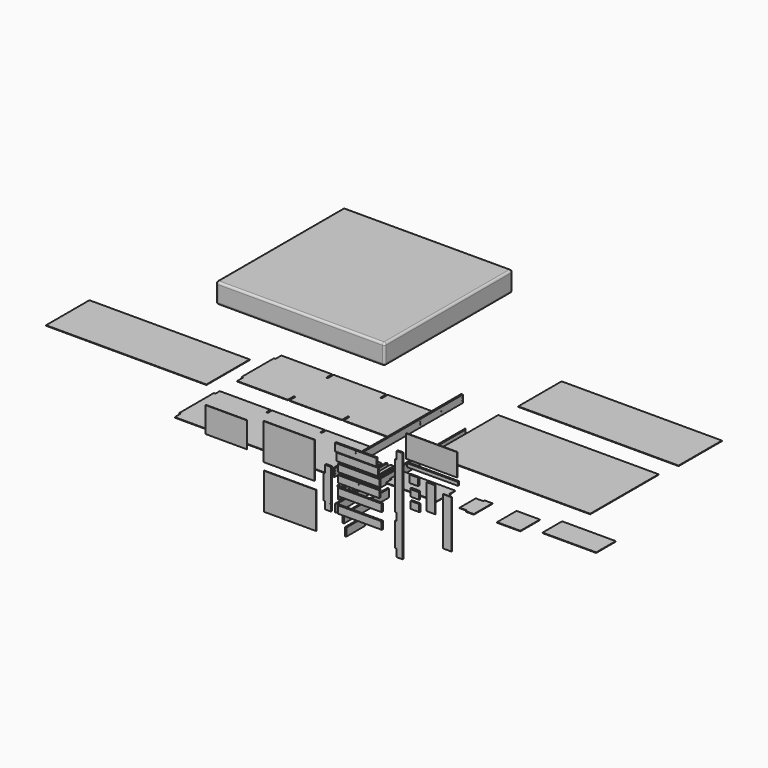
from build123d import *

# Parameters (mm, degrees)
F1_DEPTH   = 19.05
F2_D       = 6.35
F4_D       = 6.35
F4_DEPTH   = 25.4
F4_TIP     = 1.9077324654
F5_D       = 6.35
F5_DEPTH   = 25.4
F5_TIP     = 1.9077324654
F6_D       = 6.35
F6_DEPTH   = 25.4
F6_TIP     = 1.9077324654
F7_D       = 6.35
F7_DEPTH   = 25.4
F7_TIP     = 1.9077324654
F9_D       = 6.35
F9_DEPTH   = 25.4
F9_TIP     = 1.9077324654
F10_D      = 6.35
F10_DEPTH  = 25.4
F10_TIP    = 1.9077324654
F11_D      = 6.35
F11_DEPTH  = 25.4
F11_TIP    = 1.9077324654
F12_D      = 6.35
F12_DEPTH  = 25.4
F12_TIP    = 1.9077324654
F13_D      = 3.302
F13_DEPTH  = 25.4
F13_TIP    = 0.992020882
F14_D      = 3.302
F14_DEPTH  = 25.4
F14_TIP    = 0.992020882
F15_W      = 520.7
F15_H      = 88.9
F16_DEPTH  = 19.05
F17_D      = 6.35
F18_D      = 6.35
F20_D      = 6.35
F20_DEPTH  = 25.4
F20_TIP    = 1.9077324654
F21_D      = 6.35
F21_DEPTH  = 25.4
F21_TIP    = 1.9077324654
F23_D      = 6.35
F23_DEPTH  = 25.4
F23_TIP    = 1.9077324654
F24_D      = 6.35
F24_DEPTH  = 25.4
F24_TIP    = 1.9077324654
F25_D      = 6.35
F26_D      = 6.35
F27_W      = 520.7
F27_H      = 88.9
F28_DEPTH  = 19.05
F30_D      = 6.35
F30_DEPTH  = 25.4
F30_TIP    = 1.9077324654
F31_D      = 6.35
F31_DEPTH  = 25.4
F31_TIP    = 1.9077324654
F33_D      = 6.35
F33_DEPTH  = 25.4
F33_TIP    = 1.9077324654
F34_D      = 6.35
F34_DEPTH  = 25.4
F34_TIP    = 1.9077324654
F36_W      = 41.275
F36_H      = 606.425
F37_DEPTH  = 19.05
F36_H_2    = 628.65
F38_DEPTH  = 19.05
F40_D      = 6.35
F40_DEPTH  = 25.4
F40_TIP    = 1.9077324654
F41_D      = 6.35
F41_DEPTH  = 25.4
F41_TIP    = 1.9077324654
F43_D      = 6.35
F43_DEPTH  = 25.4
F43_TIP    = 1.9077324654
F44_D      = 6.35
F44_DEPTH  = 25.4
F44_TIP    = 1.9077324654
F46_D      = 6.35
F46_DEPTH  = 25.4
F46_TIP    = 1.9077324654
F47_D      = 6.35
F47_DEPTH  = 25.4
F47_TIP    = 1.9077324654
F49_D      = 6.35
F49_DEPTH  = 25.4
F49_TIP    = 1.9077324654
F50_D      = 6.35
F50_DEPTH  = 25.4
F50_TIP    = 1.9077324654
F51_W      = 1917.7
F51_H      = 88.9
F52_DEPTH  = 19.05
F53_D      = 6.35
F54_D      = 6.35
F55_D      = 3.302
F56_D      = 3.302
F57_D      = 6.35
F58_D      = 6.35
F59_D      = 6.35
F60_D      = 6.35
F61_D      = 6.35
F62_D      = 6.35
F63_D      = 3.302
F64_D      = 3.302
F65_W      = 606.425
F65_H      = 431.8
F66_DEPTH  = 6.35
F67_W      = 622.3
F67_H      = 431.8
F68_DEPTH  = 6.35
F70_DEPTH  = 6.35
F71_W      = 715.9752
F71_H      = 95.25
F72_DEPTH  = 17.4752
F73_SIZE   = 17.47519
F74_W      = 1952.6504
F74_H      = 95.25
F75_DEPTH  = 17.4752
F76_SIZE   = 17.47519
F77_SIZE   = 17.47519
F78_W      = 495.3
F78_H      = 6.35
F79_DEPTH  = 12.7
F80_W      = 495.3
F80_H      = 82.55
F81_DEPTH  = 19.05
F83_D      = 6.35
F83_DEPTH  = 25.4
F83_TIP    = 1.9077324654
F84_D      = 6.35
F84_DEPTH  = 25.4
F84_TIP    = 1.9077324654
F86_D      = 6.35
F86_DEPTH  = 25.4
F86_TIP    = 1.9077324654
F87_D      = 5.334
F88_D      = 5.334
F90_DEPTH  = 6.35
F91_W      = 673.1
F91_H      = 95.25
F92_DEPTH  = 17.4752
F93_W      = 495.3
F93_H      = 304.8
F94_DEPTH  = 6.35
F95_W      = 1917.7
F95_H      = 1022.35
F96_DEPTH  = 6.35
F98_DEPTH  = 9.525
F100_D     = 6.35
F100_DEPTH = 25.4
F100_TIP   = 1.9077324654
F101_D     = 6.35
F101_DEPTH = 25.4
F101_TIP   = 1.9077324654
F102_D     = 6.35
F102_DEPTH = 25.4
F102_TIP   = 1.9077324654
F103_W     = 101.6
F103_H     = 88.9
F104_DEPTH = 19.05
F106_D     = 6.35
F106_DEPTH = 25.4
F106_TIP   = 1.9077324654
F108_D     = 6.35
F108_DEPTH = 25.4
F108_TIP   = 1.9077324654
F109_W     = 2019.3
F109_H     = 1917.7
F110_DEPTH = 241.3
F111_R     = 25.4
F113_D     = 6.35
F113_DEPTH = 25.4
F113_TIP   = 1.9077324654
F114_D     = 6.35
F114_DEPTH = 25.4
F114_TIP   = 1.9077324654
F115_W     = 1917.7
F115_H     = 647.7
F116_DEPTH = 6.35
F118_DEPTH = 6.35
F120_DEPTH = 6.35
F121_W     = 279.4
F121_H     = 95.25
F122_DEPTH = 17.4752
F123_W     = 279.4
F123_H     = 292.1
F124_DEPTH = 6.35
F125_W     = 641.35
F125_H     = 292.1
F126_DEPTH = 6.35
F80_H_2    = 6.35
F127_DEPTH = 12.7
F78_H_2    = 82.55
F128_DEPTH = 19.05
F129_D     = 6.35
F130_D     = 6.35
F132_D     = 6.35
F132_DEPTH = 25.4
F132_TIP   = 1.9077324654
F134_D     = 6.35
F134_DEPTH = 25.4
F134_TIP   = 1.9077324654
F135_W     = 495.3
F135_H     = 88.9
F136_DEPTH = 19.05
F138_D     = 6.35
F138_DEPTH = 25.4
F138_TIP   = 1.9077324654
F140_D     = 6.35
F140_DEPTH = 25.4
F140_TIP   = 1.9077324654
F141_W     = 495.3
F141_H     = 88.9
F142_DEPTH = 19.05
F143_D     = 6.35
F144_D     = 6.35
F145_D     = 6.35
F145_DEPTH = 25.4
F145_TIP   = 1.9077324654
F147_D     = 6.35
F147_DEPTH = 25.4
F147_TIP   = 1.9077324654
F149_D     = 6.35
F149_DEPTH = 25.4
F149_TIP   = 1.9077324654
F150_W     = 101.6
F150_H     = 76.2
F151_DEPTH = 19.05
F150_H_2   = 6.35
F152_DEPTH = 12.7
F153_DEPTH = 12.7
F155_D     = 6.35
F155_DEPTH = 25.4
F155_TIP   = 1.9077324654
F157_D     = 6.35
F157_DEPTH = 25.4
F157_TIP   = 1.9077324654
F159_D     = 6.35
F159_DEPTH = 25.4
F159_TIP   = 1.9077324654
F161_D     = 6.35
F161_DEPTH = 25.4
F161_TIP   = 1.9077324654
F162_W     = 101.6
F162_H     = 82.55
F163_DEPTH = 19.05
F162_H_2   = 6.35
F164_DEPTH = 12.7
F166_D     = 6.35
F166_DEPTH = 25.4
F166_TIP   = 1.9077324654
F168_D     = 6.35
F168_DEPTH = 25.4
F168_TIP   = 1.9077324654
F169_W     = 606.425
F169_H     = 41.275
F170_DEPTH = 19.05
F172_D     = 6.35
F172_DEPTH = 25.4
F172_TIP   = 1.9077324654
F174_D     = 6.35
F174_DEPTH = 25.4
F174_TIP   = 1.9077324654
F175_W     = 606.425
F175_H     = 266.7
F176_DEPTH = 6.35
F177_W     = 101.6
F177_H     = 304.8
F178_DEPTH = 6.35
F179_W     = 101.6
F179_H     = 571.5
F180_DEPTH = 6.35
F181_W     = 1917.7
F181_H     = 647.7
F182_DEPTH = 6.35


# Not quite as in the source:
# - a fillet or chamfer is up to 0.001 mm smaller than in the source, because OpenCascade refuses the exact size
# - a feature names something its author has since deleted; it is built from what else it names


with BuildPart() as f1:
    # F0 (on Front) → F1 (new body)
    with BuildSketch(Plane.XZ):
        Polygon((44.0972222222, -217.6638888889), (44.0972222222, 252.2361111111), (-25.7527777778, 252.2361111111), (-25.7527777778, 163.3361111111), (-44.8027777778, 163.3361111111), (-44.8027777778, -128.7638888889), (-25.7527777778, -128.7638888889), (-25.7527777778, -217.6638888889), align=None)
    extrude(amount=F1_DEPTH)

    # F2 (through all)
    with Locations(Plane(origin=(0, 0, 0), x_dir=(1, 0, 0), z_dir=(0, 1, 0))):
        with Locations((36.1597222222, 138.2888888889)):
            Hole(F2_D / 2)

    # F4
    with Locations(Plane.YZ.offset(44.0972222222)):
        with Locations((-9.525, -189.0888888889)):
            Hole(F4_D / 2, depth=F4_DEPTH)
            with Locations((0, 0, -(F4_DEPTH + F4_TIP / 2))):  # 118° drill point
                Cone(0, F4_D / 2, F4_TIP, mode=Mode.SUBTRACT)

    # F5
    with Locations(Plane.YZ.offset(44.0972222222)):
        with Locations((-9.525, -157.3388888889)):
            Hole(F5_D / 2, depth=F5_DEPTH)
            with Locations((0, 0, -(F5_DEPTH + F5_TIP / 2))):  # 118° drill point
                Cone(0, F5_D / 2, F5_TIP, mode=Mode.SUBTRACT)

    # F6
    with Locations(Plane.YZ.offset(44.0972222222)):
        with Locations((-9.525, 223.6611111111)):
            Hole(F6_D / 2, depth=F6_DEPTH)
            with Locations((0, 0, -(F6_DEPTH + F6_TIP / 2))):  # 118° drill point
                Cone(0, F6_D / 2, F6_TIP, mode=Mode.SUBTRACT)

    # F7
    with Locations(Plane.YZ.offset(44.0972222222)):
        with Locations((-9.525, 191.9111111111)):
            Hole(F7_D / 2, depth=F7_DEPTH)
            with Locations((0, 0, -(F7_DEPTH + F7_TIP / 2))):  # 118° drill point
                Cone(0, F7_D / 2, F7_TIP, mode=Mode.SUBTRACT)

    # F9
    with Locations(Plane(origin=(-25.7527777778, 0, 0), x_dir=(0, -1, 0), z_dir=(-1, 0, 0))):
        with Locations((9.525, -189.0888888889)):
            Hole(F9_D / 2, depth=F9_DEPTH)
            with Locations((0, 0, -(F9_DEPTH + F9_TIP / 2))):  # 118° drill point
                Cone(0, F9_D / 2, F9_TIP, mode=Mode.SUBTRACT)

    # F10
    with Locations(Plane(origin=(-25.7527777778, 0, 0), x_dir=(0, -1, 0), z_dir=(-1, 0, 0))):
        with Locations((9.525, -157.3388888889)):
            Hole(F10_D / 2, depth=F10_DEPTH)
            with Locations((0, 0, -(F10_DEPTH + F10_TIP / 2))):  # 118° drill point
                Cone(0, F10_D / 2, F10_TIP, mode=Mode.SUBTRACT)

    # F11
    with Locations(Plane(origin=(-25.7527777778, 0, 0), x_dir=(0, -1, 0), z_dir=(-1, 0, 0))):
        with Locations((9.525, 191.9111111111)):
            Hole(F11_D / 2, depth=F11_DEPTH)
            with Locations((0, 0, -(F11_DEPTH + F11_TIP / 2))):  # 118° drill point
                Cone(0, F11_D / 2, F11_TIP, mode=Mode.SUBTRACT)

    # F12
    with Locations(Plane(origin=(-25.7527777778, 0, 0), x_dir=(0, -1, 0), z_dir=(-1, 0, 0))):
        with Locations((9.525, 223.6611111111)):
            Hole(F12_D / 2, depth=F12_DEPTH)
            with Locations((0, 0, -(F12_DEPTH + F12_TIP / 2))):  # 118° drill point
                Cone(0, F12_D / 2, F12_TIP, mode=Mode.SUBTRACT)

    # F13
    with Locations(Plane(origin=(-25.7527777778, 0, 0), x_dir=(0, -1, 0), z_dir=(-1, 0, 0))):
        with Locations((9.525, -173.2138888889)):
            Hole(F13_D / 2, depth=F13_DEPTH)
            with Locations((0, 0, -(F13_DEPTH + F13_TIP / 2))):  # 118° drill point
                Cone(0, F13_D / 2, F13_TIP, mode=Mode.SUBTRACT)

    # F14
    with Locations(Plane(origin=(-25.7527777778, 0, 0), x_dir=(0, -1, 0), z_dir=(-1, 0, 0))):
        with Locations((9.525, 207.7861111111)):
            Hole(F14_D / 2, depth=F14_DEPTH)
            with Locations((0, 0, -(F14_DEPTH + F14_TIP / 2))):  # 118° drill point
                Cone(0, F14_D / 2, F14_TIP, mode=Mode.SUBTRACT)


with BuildPart() as f16:
    # F15 (on Front) → F16 (new body)
    with BuildSketch(Plane.XZ):
        with Locations((392.2159543753, -168.203163892)):
            Rectangle(F15_W, F15_H)
    extrude(amount=F16_DEPTH)

    # F17 (through all)
    with Locations(Plane(origin=(0, 0, 0), x_dir=(1, 0, 0), z_dir=(0, 1, 0))):
        with Locations((139.8161543753, 133.278163892)):
            Hole(F17_D / 2)

    # F18 (through all)
    with Locations(Plane(origin=(0, 0, 0), x_dir=(1, 0, 0), z_dir=(0, 1, 0))):
        with Locations((644.6157543753, 133.278163892)):
            Hole(F18_D / 2)

    # F20
    with Locations(Plane.YZ.offset(652.5659543753)):
        with Locations((-9.525, -152.328163892)):
            Hole(F20_D / 2, depth=F20_DEPTH)
            with Locations((0, 0, -(F20_DEPTH + F20_TIP / 2))):  # 118° drill point
                Cone(0, F20_D / 2, F20_TIP, mode=Mode.SUBTRACT)

    # F21
    with Locations(Plane.YZ.offset(652.5659543753)):
        with Locations((-9.525, -184.078163892)):
            Hole(F21_D / 2, depth=F21_DEPTH)
            with Locations((0, 0, -(F21_DEPTH + F21_TIP / 2))):  # 118° drill point
                Cone(0, F21_D / 2, F21_TIP, mode=Mode.SUBTRACT)

    # F23
    with Locations(Plane(origin=(131.8659543753, 0, 0), x_dir=(0, -1, 0), z_dir=(-1, 0, 0))):
        with Locations((9.525, -152.328163892)):
            Hole(F23_D / 2, depth=F23_DEPTH)
            with Locations((0, 0, -(F23_DEPTH + F23_TIP / 2))):  # 118° drill point
                Cone(0, F23_D / 2, F23_TIP, mode=Mode.SUBTRACT)

    # F24
    with Locations(Plane(origin=(131.8659543753, 0, 0), x_dir=(0, -1, 0), z_dir=(-1, 0, 0))):
        with Locations((9.525, -184.078163892)):
            Hole(F24_D / 2, depth=F24_DEPTH)
            with Locations((0, 0, -(F24_DEPTH + F24_TIP / 2))):  # 118° drill point
                Cone(0, F24_D / 2, F24_TIP, mode=Mode.SUBTRACT)

    # F25 (through all)
    with Locations(Plane(origin=(0, 0, 0), x_dir=(1, 0, 0), z_dir=(0, 1, 0))):
        with Locations((392.2159543753, 136.453163892)):
            Hole(F25_D / 2)

    # F26 (through all)
    with Locations(Plane(origin=(0, 0, 0), x_dir=(1, 0, 0), z_dir=(0, 1, 0))):
        with Locations((392.2159543753, 152.328163892)):
            Hole(F26_D / 2)


with BuildPart() as f28:
    # F27 (on Front) → F28 (new body)
    with BuildSketch(Plane.XZ):
        with Locations((390.0367697954, 17.3669979692)):
            Rectangle(F27_W, F27_H)
    extrude(amount=F28_DEPTH)

    # F30
    with Locations(Plane.YZ.offset(650.3867697954)):
        with Locations((-9.525, 33.2419979692)):
            Hole(F30_D / 2, depth=F30_DEPTH)
            with Locations((0, 0, -(F30_DEPTH + F30_TIP / 2))):  # 118° drill point
                Cone(0, F30_D / 2, F30_TIP, mode=Mode.SUBTRACT)

    # F31
    with Locations(Plane.YZ.offset(650.3867697954)):
        with Locations((-9.525, 1.4919979692)):
            Hole(F31_D / 2, depth=F31_DEPTH)
            with Locations((0, 0, -(F31_DEPTH + F31_TIP / 2))):  # 118° drill point
                Cone(0, F31_D / 2, F31_TIP, mode=Mode.SUBTRACT)

    # F33
    with Locations(Plane(origin=(129.6867697954, 0, 0), x_dir=(0, -1, 0), z_dir=(-1, 0, 0))):
        with Locations((9.525, 33.2419979692)):
            Hole(F33_D / 2, depth=F33_DEPTH)
            with Locations((0, 0, -(F33_DEPTH + F33_TIP / 2))):  # 118° drill point
                Cone(0, F33_D / 2, F33_TIP, mode=Mode.SUBTRACT)

    # F34
    with Locations(Plane(origin=(129.6867697954, 0, 0), x_dir=(0, -1, 0), z_dir=(-1, 0, 0))):
        with Locations((9.525, 1.4919979692)):
            Hole(F34_D / 2, depth=F34_DEPTH)
            with Locations((0, 0, -(F34_DEPTH + F34_TIP / 2))):  # 118° drill point
                Cone(0, F34_D / 2, F34_TIP, mode=Mode.SUBTRACT)


with BuildPart() as f37:
    # F36 (on face) → F37 (new body)
    with BuildSketch(Plane.XY):
        with Locations((65.2231872082, 383.8816340816)):
            Rectangle(F36_W, F36_H)
    extrude(amount=F37_DEPTH)

    # F43
    with Locations(Plane.XZ.offset(-80.6691340816)):
        with Locations((73.1606872082, 9.525)):
            Hole(F43_D / 2, depth=F43_DEPTH)
            with Locations((0, 0, -(F43_DEPTH + F43_TIP / 2))):  # 118° drill point
                Cone(0, F43_D / 2, F43_TIP, mode=Mode.SUBTRACT)

    # F44
    with Locations(Plane.XZ.offset(-80.6691340816)):
        with Locations((57.2856872082, 9.525)):
            Hole(F44_D / 2, depth=F44_DEPTH)
            with Locations((0, 0, -(F44_DEPTH + F44_TIP / 2))):  # 118° drill point
                Cone(0, F44_D / 2, F44_TIP, mode=Mode.SUBTRACT)

    # F46
    with Locations(Plane(origin=(0, 687.0941340816, 0), x_dir=(-1, 0, 0), z_dir=(0, 1, 0))):
        with Locations((-73.1606872082, 9.525)):
            Hole(F46_D / 2, depth=F46_DEPTH)
            with Locations((0, 0, -(F46_DEPTH + F46_TIP / 2))):  # 118° drill point
                Cone(0, F46_D / 2, F46_TIP, mode=Mode.SUBTRACT)

    # F47
    with Locations(Plane(origin=(0, 687.0941340816, 0), x_dir=(-1, 0, 0), z_dir=(0, 1, 0))):
        with Locations((-57.2856872082, 9.525)):
            Hole(F47_D / 2, depth=F47_DEPTH)
            with Locations((0, 0, -(F47_DEPTH + F47_TIP / 2))):  # 118° drill point
                Cone(0, F47_D / 2, F47_TIP, mode=Mode.SUBTRACT)


with BuildPart() as f38:
    # F36 (on face) → F38 (new body)
    with BuildSketch(Plane.XY):
        with Locations((191.2130686522, 397.9515534163)):
            Rectangle(F36_W, F36_H_2)
    extrude(amount=F38_DEPTH)

    # F40
    with Locations(Plane.XZ.offset(-83.6265534163)):
        with Locations((183.2755686522, 9.525)):
            Hole(F40_D / 2, depth=F40_DEPTH)
            with Locations((0, 0, -(F40_DEPTH + F40_TIP / 2))):  # 118° drill point
                Cone(0, F40_D / 2, F40_TIP, mode=Mode.SUBTRACT)

    # F41
    with Locations(Plane.XZ.offset(-83.6265534163)):
        with Locations((199.1505686522, 9.525)):
            Hole(F41_D / 2, depth=F41_DEPTH)
            with Locations((0, 0, -(F41_DEPTH + F41_TIP / 2))):  # 118° drill point
                Cone(0, F41_D / 2, F41_TIP, mode=Mode.SUBTRACT)

    # F49
    with Locations(Plane(origin=(0, 712.2765534163, 0), x_dir=(-1, 0, 0), z_dir=(0, 1, 0))):
        with Locations((-183.2755686522, 10.0011052564)):
            Hole(F49_D / 2, depth=F49_DEPTH)
            with Locations((0, 0, -(F49_DEPTH + F49_TIP / 2))):  # 118° drill point
                Cone(0, F49_D / 2, F49_TIP, mode=Mode.SUBTRACT)

    # F50
    with Locations(Plane(origin=(0, 712.2765534163, 0), x_dir=(-1, 0, 0), z_dir=(0, 1, 0))):
        with Locations((-199.1505686522, 9.525)):
            Hole(F50_D / 2, depth=F50_DEPTH)
            with Locations((0, 0, -(F50_DEPTH + F50_TIP / 2))):  # 118° drill point
                Cone(0, F50_D / 2, F50_TIP, mode=Mode.SUBTRACT)


with BuildPart() as f52:
    # F51 (on Right) → F52 (new body)
    with BuildSketch(Plane.YZ):
        with Locations((1025.7683731079, 146.691538465)):
            Rectangle(F51_W, F51_H)
    extrude(amount=F52_DEPTH)

    # F53 (through all)
    with Locations(Plane(origin=(0, 0, 0), x_dir=(0, 1, 0), z_dir=(-1, 0, 0))):
        with Locations((76.4433731079, -162.566538465)):
            Hole(F53_D / 2)

    # F54 (through all)
    with Locations(Plane(origin=(0, 0, 0), x_dir=(0, 1, 0), z_dir=(-1, 0, 0))):
        with Locations((76.4433731079, -130.816538465)):
            Hole(F54_D / 2)

    # F55 (through all)
    with Locations(Plane(origin=(0, 0, 0), x_dir=(0, 1, 0), z_dir=(-1, 0, 0))):
        with Locations((76.4433731079, -146.691538465)):
            Hole(F55_D / 2)

    # F56 (through all)
    with Locations(Plane(origin=(0, 0, 0), x_dir=(0, 1, 0), z_dir=(-1, 0, 0))):
        with Locations((1975.0933731079, -146.691538465)):
            Hole(F56_D / 2)

    # F57 (through all)
    with Locations(Plane(origin=(0, 0, 0), x_dir=(0, 1, 0), z_dir=(-1, 0, 0))):
        with Locations((1975.0933731079, -162.566538465)):
            Hole(F57_D / 2)

    # F58 (through all)
    with Locations(Plane(origin=(0, 0, 0), x_dir=(0, 1, 0), z_dir=(-1, 0, 0))):
        with Locations((1975.0933731079, -130.816538465)):
            Hole(F58_D / 2)

    # F59 (through all)
    with Locations(Plane(origin=(0, 0, 0), x_dir=(0, 1, 0), z_dir=(-1, 0, 0))):
        with Locations((1349.6183731079, -162.566538465)):
            Hole(F59_D / 2)

    # F60 (through all)
    with Locations(Plane(origin=(0, 0, 0), x_dir=(0, 1, 0), z_dir=(-1, 0, 0))):
        with Locations((1349.6183731079, -130.816538465)):
            Hole(F60_D / 2)

    # F61 (through all)
    with Locations(Plane(origin=(0, 0, 0), x_dir=(0, 1, 0), z_dir=(-1, 0, 0))):
        with Locations((701.9183731079, -162.566538465)):
            Hole(F61_D / 2)

    # F62 (through all)
    with Locations(Plane(origin=(0, 0, 0), x_dir=(0, 1, 0), z_dir=(-1, 0, 0))):
        with Locations((701.9183731079, -130.816538465)):
            Hole(F62_D / 2)

    # F63 (through all)
    with Locations(Plane(origin=(0, 0, 0), x_dir=(0, 1, 0), z_dir=(-1, 0, 0))):
        with Locations((701.9183731079, -146.691538465)):
            Hole(F63_D / 2)

    # F64 (through all)
    with Locations(Plane(origin=(0, 0, 0), x_dir=(0, 1, 0), z_dir=(-1, 0, 0))):
        with Locations((1349.6183731079, -146.691538465)):
            Hole(F64_D / 2)

    # F87 (through all)
    with Locations(Plane(origin=(0, 0, 0), x_dir=(0, 1, 0), z_dir=(-1, 0, 0))):
        with Locations((1662.3431731079, -146.691538465)):
            Hole(F87_D / 2)

    # F88 (through all)
    with Locations(Plane(origin=(0, 0, 0), x_dir=(0, 1, 0), z_dir=(-1, 0, 0))):
        with Locations((389.1808731079, -146.691538465)):
            Hole(F88_D / 2)


with BuildPart() as f66:
    # F65 (on Front) → F66 (new body)
    with BuildSketch(Plane.XZ):
        with Locations((-466.6956380844, 248.3464175232)):
            Rectangle(F65_W, F65_H)
    extrude(amount=F66_DEPTH)


with BuildPart() as f68:
    # F67 (on face) → F68 (new body)
    with BuildSketch(Plane.XZ.offset(6.35)):
        with Locations((-450.0797018051, -268.8254054308)):
            Rectangle(F67_W, F67_H)
    extrude(amount=F68_DEPTH)


with BuildPart() as f70:
    # F69 (on Top) → F70 (new body)
    with BuildSketch(Plane.XY):
        Polygon((-1412.1244818761, 898.8181884059), (-2018.5494818761, 898.8181884059), (-2018.5494818761, 835.3181884059), (-2037.5994818761, 835.3181884059), (-2037.5994818761, 314.6181884059), (-2018.5494818761, 314.6181884059), (-2018.5494818761, 225.7181884059), (-1412.1244818761, 225.7181884059), (-1412.1244818761, 314.6181884059), (-1393.0744818761, 314.6181884059), (-1393.0744818761, 225.7181884059), (-764.4244818761, 225.7181884059), (-764.4244818761, 314.6181884059), (-745.3744818761, 314.6181884059), (-745.3744818761, 225.7181884059), (-138.9494818761, 225.7181884059), (-138.9494818761, 314.6181884059), (-119.8994818761, 314.6181884059), (-119.8994818761, 835.3181884059), (-138.9494818761, 835.3181884059), (-138.9494818761, 898.8181884059), (-745.3744818761, 898.8181884059), (-745.3744818761, 835.3181884059), (-764.4244818761, 835.3181884059), (-764.4244818761, 898.8181884059), (-1393.0744818761, 898.8181884059), (-1393.0744818761, 835.3181884059), (-1412.1244818761, 835.3181884059), align=None)
    extrude(amount=F70_DEPTH)


with BuildPart() as f72:
    # F71 (on Right) → F72 (new body)
    with BuildSketch(Plane.YZ):
        with Locations((501.9332787514, -122.720502317)):
            Rectangle(F71_W, F71_H)
    extrude(amount=F72_DEPTH)

    # F73 (size 17.4752 in the source; OpenCascade refuses exactly that, so slightly less here)
    f73_edges = [f72.edges().sort_by_distance(p)[0] for p in [
        (17.4752, 143.945679, -122.720502),
    ]]
    chamfer(f73_edges, length=F73_SIZE)


with BuildPart() as f75:
    # F74 (on Right) → F75 (new body)
    with BuildSketch(Plane.YZ):
        with Locations((1071.8703280807, -243.98250422)):
            Rectangle(F74_W, F74_H)
    extrude(amount=F75_DEPTH)

    # F76 (size 17.4752 in the source; OpenCascade refuses exactly that, so slightly less here)
    f76_edges = [f75.edges().sort_by_distance(p)[0] for p in [
        (17.4752, 95.545128, -243.982504),
    ]]
    chamfer(f76_edges, length=F76_SIZE)

    # F77 (size 17.4752 in the source; OpenCascade refuses exactly that, so slightly less here)
    f77_edges = [f75.edges().sort_by_distance(p)[0] for p in [
        (17.4752, 2048.195528, -243.982504),
    ]]
    chamfer(f77_edges, length=F77_SIZE)


with BuildPart() as f79:
    # F78 (on Front) → F79 (new body)
    with BuildSketch(Plane.XZ):
        with Locations((375.5939779373, 197.4594274402)):
            Rectangle(F78_W, F78_H)
    extrude(amount=F79_DEPTH)

    # F78 (on Front) → F128 (join)
    with BuildSketch(Plane.XZ):
        with Locations((375.5939779373, 153.0094274402)):
            Rectangle(F78_W, F78_H_2)
    extrude(amount=F128_DEPTH)

    # F129 (through all)
    with Locations(Plane(origin=(0, 0, 0), x_dir=(1, 0, 0), z_dir=(0, 1, 0))):
        with Locations((375.5939779373, -187.9344274402)):
            Hole(F129_D / 2)

    # F130 (through all)
    with Locations(Plane(origin=(0, 0, 0), x_dir=(1, 0, 0), z_dir=(0, 1, 0))):
        with Locations((375.5939779373, -172.0594274402)):
            Hole(F130_D / 2)

    # F132
    with Locations(Plane(origin=(127.9439779373, 0, 0), x_dir=(0, -1, 0), z_dir=(-1, 0, 0))):
        with Locations((9.525, 172.0594274402), (9.525, 140.3094274402)):
            Hole(F132_D / 2, depth=F132_DEPTH)
            with Locations((0, 0, -(F132_DEPTH + F132_TIP / 2))):  # 118° drill point
                Cone(0, F132_D / 2, F132_TIP, mode=Mode.SUBTRACT)

    # F134
    with Locations(Plane.YZ.offset(623.2439779373)):
        with Locations((-9.525, 172.0594274402), (-9.525, 140.3094274402)):
            Hole(F134_D / 2, depth=F134_DEPTH)
            with Locations((0, 0, -(F134_DEPTH + F134_TIP / 2))):  # 118° drill point
                Cone(0, F134_D / 2, F134_TIP, mode=Mode.SUBTRACT)


with BuildPart() as f81:
    # F80 (on Front) → F81 (new body)
    with BuildSketch(Plane.XZ):
        with Locations((375.3500119215, 270.1343170285)):
            Rectangle(F80_W, F80_H)
    extrude(amount=F81_DEPTH)

    # F83
    with Locations(Plane(origin=(127.7000119215, 0, 0), x_dir=(0, -1, 0), z_dir=(-1, 0, 0))):
        with Locations((9.525, 282.8343170285)):
            Hole(F83_D / 2, depth=F83_DEPTH)
            with Locations((0, 0, -(F83_DEPTH + F83_TIP / 2))):  # 118° drill point
                Cone(0, F83_D / 2, F83_TIP, mode=Mode.SUBTRACT)

    # F84
    with Locations(Plane(origin=(127.7000119215, 0, 0), x_dir=(0, -1, 0), z_dir=(-1, 0, 0))):
        with Locations((9.525, 251.0843170285)):
            Hole(F84_D / 2, depth=F84_DEPTH)
            with Locations((0, 0, -(F84_DEPTH + F84_TIP / 2))):  # 118° drill point
                Cone(0, F84_D / 2, F84_TIP, mode=Mode.SUBTRACT)

    # F86
    with Locations(Plane.YZ.offset(623.0000119215)):
        with Locations((-9.525, 282.8343170285)):
            Hole(F86_D / 2, depth=F86_DEPTH)
            with Locations((0, 0, -(F86_DEPTH + F86_TIP / 2))):  # 118° drill point
                Cone(0, F86_D / 2, F86_TIP, mode=Mode.SUBTRACT)

    # F80 (on Front) → F127 (join)
    with BuildSketch(Plane.XZ):
        with Locations((375.3500119215, 225.6843170285)):
            Rectangle(F80_W, F80_H_2)
    extrude(amount=F127_DEPTH)

    # F145
    with Locations(Plane.YZ.offset(623.0000119215)):
        with Locations((-9.525, 251.0843170285)):
            Hole(F145_D / 2, depth=F145_DEPTH)
            with Locations((0, 0, -(F145_DEPTH + F145_TIP / 2))):  # 118° drill point
                Cone(0, F145_D / 2, F145_TIP, mode=Mode.SUBTRACT)


with BuildPart() as f90:
    # F89 (on Top) → F90 (new body)
    with BuildSketch(Plane.XY):
        Polygon((-1412.908935664, 1820.1076601933), (-2019.333935664, 1820.1076601933), (-2019.333935664, 1731.2076601933), (-2038.383935664, 1731.2076601933), (-2038.383935664, 1248.6076601933), (-2019.333935664, 1248.6076601933), (-2019.333935664, 1159.7076601933), (-1412.908935664, 1159.7076601933), (-1412.908935664, 1248.6076601933), (-1393.858935664, 1248.6076601933), (-1393.858935664, 1159.7076601933), (-765.208935664, 1159.7076601933), (-765.208935664, 1248.6076601933), (-746.158935664, 1248.6076601933), (-746.158935664, 1159.7076601933), (-139.733935664, 1159.7076601933), (-139.733935664, 1248.6076601933), (-120.683935664, 1248.6076601933), (-120.683935664, 1731.2076601933), (-139.733935664, 1731.2076601933), (-139.733935664, 1820.1076601933), (-746.158935664, 1820.1076601933), (-746.158935664, 1731.2076601933), (-765.208935664, 1731.2076601933), (-765.208935664, 1820.1076601933), (-1393.858935664, 1820.1076601933), (-1393.858935664, 1731.2076601933), (-1412.908935664, 1731.2076601933), align=None)
    extrude(amount=F90_DEPTH)


with BuildPart() as f92:
    # F91 (on Right) → F92 (new body)
    with BuildSketch(Plane.YZ):
        with Locations((547.2309960085, -398.1397897005)):
            Rectangle(F91_W, F91_H)
    extrude(amount=F92_DEPTH)


with BuildPart() as f94:
    # F93 (on Front) → F94 (new body)
    with BuildSketch(Plane.XZ):
        with Locations((-1218.936782995, 254.6093458474)):
            Rectangle(F93_W, F93_H)
    extrude(amount=F94_DEPTH)


with BuildPart() as f96:
    # F95 (on face) → F96 (new body)
    with BuildSketch(Plane.XY.offset(6.35)):
        with Locations((1280.6541621685, 1624.7996635968)):
            Rectangle(F95_W, F95_H)
    extrude(amount=F96_DEPTH)


with BuildPart() as f98:
    # F97 (on Front) → F98 (new body, symmetric)
    with BuildSketch(Plane.XZ):
        Polygon((823.0462499619, -359.8734816171), (823.0462499619, -448.7734816171), (892.8962499619, -448.7734816171), (892.8962499619, 668.8265183829), (823.0462499619, 668.8265183829), (823.0462499619, 579.9265183829), (803.9962499619, 579.9265183829), (803.9962499619, 478.3265183829), (803.9962499619, 389.4265183829), (803.9962499619, 21.1265183829), (823.0462499619, 21.1265183829), (823.0462499619, -67.7734816171), (803.9962499619, -67.7734816171), (803.9962499619, -359.8734816171), align=None)
    extrude(amount=F98_DEPTH, both=True)

    # F100
    with Locations(Plane.YZ.offset(892.8962499619)):
        with Locations((0, -420.1984816171)):
            Hole(F100_D / 2, depth=F100_DEPTH)
            with Locations((0, 0, -(F100_DEPTH + F100_TIP / 2))):  # 118° drill point
                Cone(0, F100_D / 2, F100_TIP, mode=Mode.SUBTRACT)

    # F101
    with Locations(Plane.YZ.offset(892.8962499619)):
        with Locations((0, -388.4484816171)):
            Hole(F101_D / 2, depth=F101_DEPTH)
            with Locations((0, 0, -(F101_DEPTH + F101_TIP / 2))):  # 118° drill point
                Cone(0, F101_D / 2, F101_TIP, mode=Mode.SUBTRACT)

    # F102
    with Locations(Plane.YZ.offset(892.8962499619)):
        with Locations((0, -7.4484816171), (0, -39.1984816171)):
            Hole(F102_D / 2, depth=F102_DEPTH)
            with Locations((0, 0, -(F102_DEPTH + F102_TIP / 2))):  # 118° drill point
                Cone(0, F102_D / 2, F102_TIP, mode=Mode.SUBTRACT)

    # F113
    with Locations(Plane(origin=(823.0462499619, 0, 0), x_dir=(0, -1, 0), z_dir=(-1, 0, 0))):
        with Locations((0, 640.2515183829), (0, 608.5015183829)):
            Hole(F113_D / 2, depth=F113_DEPTH)
            with Locations((0, 0, -(F113_DEPTH + F113_TIP / 2))):  # 118° drill point
                Cone(0, F113_D / 2, F113_TIP, mode=Mode.SUBTRACT)

    # F114
    with Locations(Plane.YZ.offset(892.8962499619)):
        with Locations((0, 640.2515183829), (0, 608.5015183829)):
            Hole(F114_D / 2, depth=F114_DEPTH)
            with Locations((0, 0, -(F114_DEPTH + F114_TIP / 2))):  # 118° drill point
                Cone(0, F114_D / 2, F114_TIP, mode=Mode.SUBTRACT)

    # F159
    with Locations(Plane(origin=(823.0462499619, 0, 0), x_dir=(0, -1, 0), z_dir=(-1, 0, 0))):
        with Locations((0, -7.4484816171), (0, -39.1984816171)):
            Hole(F159_D / 2, depth=F159_DEPTH)
            with Locations((0, 0, -(F159_DEPTH + F159_TIP / 2))):  # 118° drill point
                Cone(0, F159_D / 2, F159_TIP, mode=Mode.SUBTRACT)

    # F161
    with Locations(Plane(origin=(823.0462499619, 0, 0), x_dir=(0, -1, 0), z_dir=(-1, 0, 0))):
        with Locations((0, -388.4484816171), (0, -420.1984816171)):
            Hole(F161_D / 2, depth=F161_DEPTH)
            with Locations((0, 0, -(F161_DEPTH + F161_TIP / 2))):  # 118° drill point
                Cone(0, F161_D / 2, F161_TIP, mode=Mode.SUBTRACT)


with BuildPart() as f104:
    # F103 (on face) → F104 (new body)
    with BuildSketch(Plane.XZ.offset(9.525)):
        with Locations((1043.4946498871, 439.289823246)):
            Rectangle(F103_W, F103_H)
    extrude(amount=F104_DEPTH)

    # F106
    with Locations(Plane.YZ.offset(1094.2946498871)):
        with Locations((-19.05, 455.164823246), (-19.05, 423.414823246)):
            Hole(F106_D / 2, depth=F106_DEPTH)
            with Locations((0, 0, -(F106_DEPTH + F106_TIP / 2))):  # 118° drill point
                Cone(0, F106_D / 2, F106_TIP, mode=Mode.SUBTRACT)

    # F108
    with Locations(Plane(origin=(992.6946498871, 0, 0), x_dir=(0, -1, 0), z_dir=(-1, 0, 0))):
        with Locations((19.05, 455.164823246), (19.05, 423.414823246)):
            Hole(F108_D / 2, depth=F108_DEPTH)
            with Locations((0, 0, -(F108_DEPTH + F108_TIP / 2))):  # 118° drill point
                Cone(0, F108_D / 2, F108_TIP, mode=Mode.SUBTRACT)


with BuildPart() as f110:
    # F109 (on Top) → F110 (new body)
    with BuildSketch(Plane.XY):
        with Locations((-2145.1758291454, 3216.1710262299)):
            Rectangle(F109_W, F109_H)
    extrude(amount=F110_DEPTH)

    # F111
    f111_edges = [f110.edges().sort_by_distance(p)[0] for p in [
        (-2145.175829, 2257.321026, 241.3),
        (-3154.825829, 2257.321026, 120.65),
        (-3154.825829, 3216.171026, 241.3),
        (-2145.175829, 2257.321026, 0),
        (-3154.825829, 3216.171026, 0),
        (-1135.525829, 2257.321026, 120.65),
        (-1135.525829, 3216.171026, 241.3),
        (-1135.525829, 3216.171026, 0),
        (-1135.525829, 4175.021026, 120.65),
        (-2145.175829, 4175.021026, 241.3),
        (-3154.825829, 4175.021026, 120.65),
        (-2145.175829, 4175.021026, 0),
    ]]
    fillet(f111_edges, radius=F111_R)


with BuildPart() as f116:
    # F115 (on face) → F116 (new body)
    with BuildSketch(Plane.XY.offset(12.7)):
        with Locations((1324.3790087512, 2704.3896711349)):
            Rectangle(F115_W, F115_H)
    extrude(amount=F116_DEPTH)


with BuildPart() as f118:
    # F117 (on Top) → F118 (new body)
    with BuildSketch(Plane.XY):
        Polygon((954.666505909, 701.1590391636), (348.241505909, 701.1590391636), (348.241505909, 612.2590391636), (329.191505909, 612.2590391636), (329.191505909, 510.6590391636), (348.241505909, 510.6590391636), (348.241505909, 421.7590391636), (954.666505909, 421.7590391636), (954.666505909, 510.6590391636), (973.716505909, 510.6590391636), (973.716505909, 612.2590391636), (954.666505909, 612.2590391636), align=None)
    extrude(amount=F118_DEPTH)


with BuildPart() as f120:
    # F119 (on face) → F120 (new body)
    with BuildSketch(Plane.XY.offset(6.35)):
        Polygon((1394.9772543545, 707.9822912931), (1299.7272543545, 707.9822912931), (1299.7272543545, 688.9322912931), (1210.8272543545, 688.9322912931), (1210.8272543545, 447.6322912931), (1299.7272543545, 447.6322912931), (1299.7272543545, 428.5822912931), (1394.9772543545, 428.5822912931), align=None)
    extrude(amount=F120_DEPTH)


with BuildPart() as f122:
    # F121 (on face) → F122 (new body)
    with BuildSketch(Plane.YZ.offset(17.4752)):
        with Locations((362.692411232, -536.618118763)):
            Rectangle(F121_W, F121_H)
    extrude(amount=F122_DEPTH)


with BuildPart() as f124:
    # F123 (on face) → F124 (new body)
    with BuildSketch(Plane.XY.offset(12.7)):
        with Locations((1813.7959793091, 573.3920572281)):
            Rectangle(F123_W, F123_H)
    extrude(amount=F124_DEPTH)


with BuildPart() as f126:
    # F125 (on face) → F126 (new body)
    with BuildSketch(Plane.XY.offset(19.05)):
        with Locations((2465.9060394287, 665.3391359329)):
            Rectangle(F125_W, F125_H)
    extrude(amount=F126_DEPTH)


with BuildPart() as f136:
    # F135 (on face) → F136 (new body)
    with BuildSketch(Plane.XZ.offset(19.05)):
        with Locations((372.6696048737, 393.4240490913)):
            Rectangle(F135_W, F135_H)
    extrude(amount=F136_DEPTH)

    # F138
    with Locations(Plane(origin=(125.0196048737, 0, 0), x_dir=(0, -1, 0), z_dir=(-1, 0, 0))):
        with Locations((28.575, 409.2990490913), (28.575, 377.5490490913)):
            Hole(F138_D / 2, depth=F138_DEPTH)
            with Locations((0, 0, -(F138_DEPTH + F138_TIP / 2))):  # 118° drill point
                Cone(0, F138_D / 2, F138_TIP, mode=Mode.SUBTRACT)

    # F140
    with Locations(Plane.YZ.offset(620.3196048737)):
        with Locations((-28.575, 409.2990490913), (-28.575, 377.5490490913)):
            Hole(F140_D / 2, depth=F140_DEPTH)
            with Locations((0, 0, -(F140_DEPTH + F140_TIP / 2))):  # 118° drill point
                Cone(0, F140_D / 2, F140_TIP, mode=Mode.SUBTRACT)


with BuildPart() as f142:
    # F141 (on face) → F142 (new body)
    with BuildSketch(Plane.XZ.offset(38.1)):
        with Locations((371.7590843201, 502.6594550133)):
            Rectangle(F141_W, F141_H)
    extrude(amount=F142_DEPTH)

    # F143 (through all)
    with Locations(Plane(origin=(0, -38.1, 0), x_dir=(1, 0, 0), z_dir=(0, 1, 0))):
        with Locations((371.7590843201, -534.4094550133)):
            Hole(F143_D / 2)

    # F144 (through all)
    with Locations(Plane(origin=(0, -38.1, 0), x_dir=(1, 0, 0), z_dir=(0, 1, 0))):
        with Locations((371.7590843201, -518.5344550133)):
            Hole(F144_D / 2)

    # F147
    with Locations(Plane.YZ.offset(619.4090843201)):
        with Locations((-47.625, 518.5344550133), (-47.625, 486.7844550133)):
            Hole(F147_D / 2, depth=F147_DEPTH)
            with Locations((0, 0, -(F147_DEPTH + F147_TIP / 2))):  # 118° drill point
                Cone(0, F147_D / 2, F147_TIP, mode=Mode.SUBTRACT)

    # F149
    with Locations(Plane(origin=(124.1090843201, 0, 0), x_dir=(0, -1, 0), z_dir=(-1, 0, 0))):
        with Locations((47.625, 518.5344550133), (47.625, 486.7844550133)):
            Hole(F149_D / 2, depth=F149_DEPTH)
            with Locations((0, 0, -(F149_DEPTH + F149_TIP / 2))):  # 118° drill point
                Cone(0, F149_D / 2, F149_TIP, mode=Mode.SUBTRACT)


with BuildPart() as f151:
    # F150 (on Front) → F151 (new body)
    with BuildSketch(Plane.XZ):
        with Locations((1044.4987670898, 289.0409827948)):
            Rectangle(F150_W, F150_H)
    extrude(amount=F151_DEPTH)

    # F150 (on Front) → F152 (join)
    with BuildSketch(Plane.XZ):
        with Locations((1044.4987670898, 330.3159827948)):
            Rectangle(F150_W, F150_H_2)
    extrude(amount=F152_DEPTH)

    # F150 (on Front) → F153 (join)
    with BuildSketch(Plane.XZ):
        with Locations((1044.4987670898, 247.7659827948)):
            Rectangle(F150_W, F150_H_2)
    extrude(amount=F153_DEPTH)

    # F155
    with Locations(Plane.YZ.offset(1095.2987670898)):
        with Locations((-9.525, 304.9159827948), (-9.525, 273.1659827948)):
            Hole(F155_D / 2, depth=F155_DEPTH)
            with Locations((0, 0, -(F155_DEPTH + F155_TIP / 2))):  # 118° drill point
                Cone(0, F155_D / 2, F155_TIP, mode=Mode.SUBTRACT)

    # F157
    with Locations(Plane(origin=(993.6987670898, 0, 0), x_dir=(0, -1, 0), z_dir=(-1, 0, 0))):
        with Locations((9.525, 304.9159827948), (9.525, 273.1659827948)):
            Hole(F157_D / 2, depth=F157_DEPTH)
            with Locations((0, 0, -(F157_DEPTH + F157_TIP / 2))):  # 118° drill point
                Cone(0, F157_D / 2, F157_TIP, mode=Mode.SUBTRACT)


with BuildPart() as f163:
    # F162 (on Front) → F163 (new body)
    with BuildSketch(Plane.XZ):
        with Locations((1047.939027977, 163.0283616185)):
            Rectangle(F162_W, F162_H)
    extrude(amount=F163_DEPTH)

    # F162 (on Front) → F164 (join)
    with BuildSketch(Plane.XZ):
        with Locations((1047.939027977, 118.5783616185)):
            Rectangle(F162_W, F162_H_2)
    extrude(amount=F164_DEPTH)

    # F166
    with Locations(Plane.YZ.offset(1098.739027977)):
        with Locations((-9.525, 175.7283616185), (-9.525, 143.9783616185)):
            Hole(F166_D / 2, depth=F166_DEPTH)
            with Locations((0, 0, -(F166_DEPTH + F166_TIP / 2))):  # 118° drill point
                Cone(0, F166_D / 2, F166_TIP, mode=Mode.SUBTRACT)

    # F168
    with Locations(Plane(origin=(997.139027977, 0, 0), x_dir=(0, -1, 0), z_dir=(-1, 0, 0))):
        with Locations((9.525, 175.7283616185), (9.525, 143.9783616185)):
            Hole(F168_D / 2, depth=F168_DEPTH)
            with Locations((0, 0, -(F168_DEPTH + F168_TIP / 2))):  # 118° drill point
                Cone(0, F168_D / 2, F168_TIP, mode=Mode.SUBTRACT)


with BuildPart() as f170:
    # F169 (on Front) → F170 (new body)
    with BuildSketch(Plane.XZ):
        with Locations((1260.3922124863, 567.2860619545)):
            Rectangle(F169_W, F169_H)
    extrude(amount=F170_DEPTH)

    # F172
    with Locations(Plane.YZ.offset(1563.6047124863)):
        with Locations((-9.525, 575.2235619545), (-9.525, 559.3485619545)):
            Hole(F172_D / 2, depth=F172_DEPTH)
            with Locations((0, 0, -(F172_DEPTH + F172_TIP / 2))):  # 118° drill point
                Cone(0, F172_D / 2, F172_TIP, mode=Mode.SUBTRACT)

    # F174
    with Locations(Plane(origin=(957.1797124863, 0, 0), x_dir=(0, -1, 0), z_dir=(-1, 0, 0))):
        with Locations((9.525, 575.2235619545), (9.525, 559.3485619545)):
            Hole(F174_D / 2, depth=F174_DEPTH)
            with Locations((0, 0, -(F174_DEPTH + F174_TIP / 2))):  # 118° drill point
                Cone(0, F174_D / 2, F174_TIP, mode=Mode.SUBTRACT)


with BuildPart() as f176:
    # F175 (on face) → F176 (new body)
    with BuildSketch(Plane.XZ.offset(19.05)):
        with Locations((1253.4554962158, 768.6192842484)):
            Rectangle(F175_W, F175_H)
    extrude(amount=F176_DEPTH)


with BuildPart() as f178:
    # F177 (on face) → F178 (new body)
    with BuildSketch(Plane.XZ.offset(25.4)):
        with Locations((1251.7871515274, 319.8676537514)):
            Rectangle(F177_W, F177_H)
    extrude(amount=F178_DEPTH)


with BuildPart() as f180:
    # F179 (on face) → F180 (new body)
    with BuildSketch(Plane.XZ.offset(31.75)):
        with Locations((1452.0719647408, 128.2776150824)):
            Rectangle(F179_W, F179_H)
    extrude(amount=F180_DEPTH)


with BuildPart() as f182:
    # F181 (on face) → F182 (new body)
    with BuildSketch(Plane.XY.offset(6.35)):
        with Locations((-3151.4647268295, 1240.3665424347)):
            Rectangle(F181_W, F181_H)
    extrude(amount=F182_DEPTH)


solid = Compound([f1.part, f16.part, f28.part, f37.part, f38.part, f52.part, f66.part, f68.part, f70.part, f72.part, f75.part, f79.part, f81.part, f90.part, f92.part, f94.part, f96.part, f98.part, f104.part, f110.part, f116.part, f118.part, f120.part, f122.part, f124.part, f126.part, f136.part, f142.part, f151.part, f163.part, f170.part, f176.part, f178.part, f180.part, f182.part])
